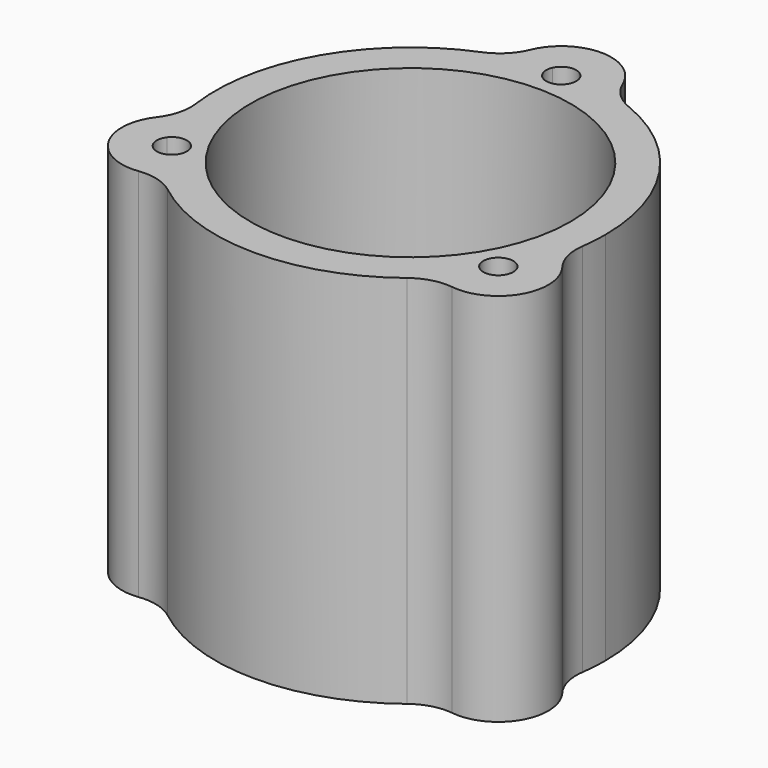
from build123d import *

# Parameters (mm, degrees)
F0_R     = 20.32
F1_DEPTH = 47.625
F2_R     = 6.35


with BuildPart() as f1:
    # F0 (on Top) → F1 (new body)
    with BuildSketch(Plane.XY):
        with BuildLine():
            ThreePointArc((23.9050999455, -6.4692674698), (24.5490837421, -3.2630832697), (24.765, 0))
            ThreePointArc((24.765, 0), (19.6285885254, 15.1004548773), (6.35, 23.9370575677))
            ThreePointArc((6.35, 23.9370575677), (4.0651088886, 24.4290833787), (1.7440091422, 24.703515076))
            ThreePointArc((1.7440091422, 24.703515076), (1.8643178935, 24.3286489263), (1.905, 23.9370575677))
            ThreePointArc((1.905, 23.9370575677), (-0.3915913586, 22.0727396742), (-1.7440091422, 24.703515076))
            ThreePointArc((-1.7440091422, 24.703515076), (-4.0651088886, 24.4290833787), (-6.35, 23.9370575677))
            ThreePointArc((-6.35, 23.9370575677), (-21.4471191247, 12.3825), (-23.9050999455, -6.4692674698))
            ThreePointArc((-23.9050999455, -6.4692674698), (-23.1887612414, -8.6940541227), (-22.2658761897, -10.8414013165))
            ThreePointArc((-22.2658761897, -10.8414013165), (-20.1370690632, -10.1581864481), (-18.8250999455, -11.9685287839))
            ThreePointArc((-18.8250999455, -11.9685287839), (-19.3113489683, -13.239815795), (-20.5218670475, -13.8621137596))
            ThreePointArc((-20.5218670475, -13.8621137596), (-19.1236523528, -15.735029256), (-17.5550999455, -17.4677900979))
            ThreePointArc((-17.5550999455, -17.4677900979), (0, -24.765), (17.5550999455, -17.4677900979))
            ThreePointArc((17.5550999455, -17.4677900979), (19.1236523528, -15.735029256), (20.5218670475, -13.8621137596))
            ThreePointArc((20.5218670475, -13.8621137596), (19.0803215513, -11.0160287839), (22.2658761897, -10.8414013165))
            ThreePointArc((22.2658761897, -10.8414013165), (23.1887612414, -8.6940541227), (23.9050999455, -6.4692674698))
        make_face()
        Circle(F0_R, mode=Mode.SUBTRACT)
        with BuildLine():
            ThreePointArc((-22.2658761897, -10.8414013165), (-23.1887612414, -8.6940541227), (-23.9050999455, -6.4692674698))
            ThreePointArc((-23.9050999455, -6.4692674698), (-26.2293612595, -15.1435287839), (-17.5550999455, -17.4677900979))
            ThreePointArc((-17.5550999455, -17.4677900979), (-19.1236523528, -15.735029256), (-20.5218670475, -13.8621137596))
            ThreePointArc((-20.5218670475, -13.8621137596), (-22.3798783397, -12.9210287839), (-22.2658761897, -10.8414013165))
        make_face()
        with BuildLine():
            ThreePointArc((1.7440091422, 24.703515076), (4.0651088886, 24.4290833787), (6.35, 23.9370575677))
            ThreePointArc((6.35, 23.9370575677), (0, 30.2870575677), (-6.35, 23.9370575677))
            ThreePointArc((-6.35, 23.9370575677), (-4.0651088886, 24.4290833787), (-1.7440091422, 24.703515076))
            ThreePointArc((-1.7440091422, 24.703515076), (0, 25.8420575677), (1.7440091422, 24.703515076))
        make_face()
        with BuildLine():
            ThreePointArc((17.5550999455, -17.4677900979), (26.2293612595, -15.1435287839), (23.9050999455, -6.4692674698))
            ThreePointArc((23.9050999455, -6.4692674698), (23.1887612414, -8.6940541227), (22.2658761897, -10.8414013165))
            ThreePointArc((22.2658761897, -10.8414013165), (22.5404422812, -11.3754979015), (22.6350999455, -11.9685287839))
            ThreePointArc((22.6350999455, -11.9685287839), (22.0013869566, -13.3872797611), (20.5218670475, -13.8621137596))
            ThreePointArc((20.5218670475, -13.8621137596), (19.1236523528, -15.735029256), (17.5550999455, -17.4677900979))
        make_face()
    extrude(amount=F1_DEPTH)

    # F2
    f2_edges = [f1.edges().sort_by_distance(p)[0] for p in [
        (6.35, 23.937058, 23.8125),
        (-23.9051, -6.469267, 23.8125),
        (17.5551, -17.46779, 23.8125),
        (23.9051, -6.469267, 23.8125),
        (-6.35, 23.937058, 23.8125),
        (-17.5551, -17.46779, 23.8125),
    ]]
    fillet(f2_edges, radius=F2_R)


solid = f1.part
